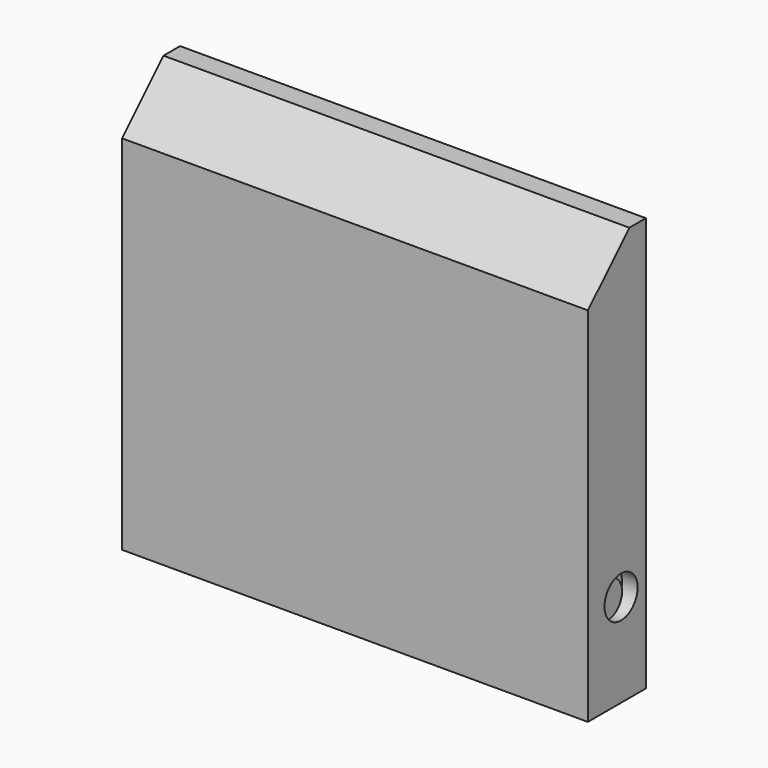
from build123d import *

# Parameters (mm, degrees)
F0_W         = 41
F0_H         = 30
F1_DEPTH     = 6
F2_T         = -2
F3_W         = 2
F3_H         = 2
F4_DEPTH     = 10
F5_R         = 1.75
F6_DEPTH     = 1
F7_R         = 1.75
F8_DEPTH     = 1
F9_W         = 45
F9_H         = 40
F10_DEPTH    = 7
F11_SIZE     = 5
F12_T        = -1.5
F13_T1_DEPTH = 66.7168298797
F16_DEPTH    = 1.5
F17_R        = 2
F18_DEPTH    = 25
F19_R        = 2
F20_DEPTH    = 25
F21_DEPTH    = 2
F22_W        = 14
F22_H        = 12
F22_W_2      = 2
F22_H_2      = 2
F23_DEPTH    = 8


# Not quite as in the source:
# - a fillet or chamfer that OpenCascade refuses, or shapes differently, is made with other operations: its cross-section is extruded or revolved along the edge and cut away or added
# - a feature names something its author has since deleted; it is built from what else it names


with BuildPart() as f1:
    # F0 (on Front) → F1 (new body)
    with BuildSketch(Plane.XZ):
        with Locations((0.5, 0)):
            Rectangle(F0_W, F0_H)
    extrude(amount=F1_DEPTH)

    # F2
    f2_openings = [f1.faces().sort_by_distance(p)[0] for p in [
        (0.5, -6, 0),
    ]]
    offset(amount=F2_T, openings=f2_openings)

    # F3 (on face) → F4 (cut)
    with BuildSketch(Plane.XZ):
        with Locations((-3, -2)):
            Rectangle(F3_W, F3_H)
        with Locations((3, -2)):
            Rectangle(F3_W, F3_H)
        with Locations((3, 2)):
            Rectangle(F3_W, F3_H)
        with Locations((-3, 2)):
            Rectangle(F3_W, F3_H)
    extrude(amount=F4_DEPTH, mode=Mode.SUBTRACT)

    # F5 (on face) → F6 (join)
    with BuildSketch(Plane.YZ.offset(21)):
        with Locations((-4, -11)):
            Circle(F5_R)
    extrude(amount=F6_DEPTH)

    # F7 (on face) → F8 (join)
    with BuildSketch(Plane(origin=(-20, 0, 0), x_dir=(0, -1, 0), z_dir=(-1, 0, 0))):
        with Locations((4, -11)):
            Circle(F7_R)
    extrude(amount=F8_DEPTH)

    # F13: chamfer of 5 on 1 edges, made by hand

    # F13_s2 → F13_t1 (cut)
    with BuildSketch(Plane.YZ.offset(-32.8584149398)):
        Polygon((-1, 15), (-6, 10), (-6, 15), align=None)
    extrude(amount=F13_T1_DEPTH, mode=Mode.SUBTRACT)

    # F22 (on face) → F23 (join)
    with BuildSketch(Plane.XZ.offset(2)):
        Rectangle(F22_W, F22_H)
        with Locations((-3, -2)):
            Rectangle(F22_W_2, F22_H_2, mode=Mode.SUBTRACT)
        with Locations((3, -2)):
            Rectangle(F22_W_2, F22_H_2, mode=Mode.SUBTRACT)
        with Locations((-3, 2)):
            Rectangle(F22_W_2, F22_H_2, mode=Mode.SUBTRACT)
        with Locations((3, 2)):
            Rectangle(F22_W_2, F22_H_2, mode=Mode.SUBTRACT)
    extrude(amount=-F23_DEPTH)


with BuildPart() as f10:
    # F9 (on Front) → F10 (new body)
    with BuildSketch(Plane.XZ):
        Rectangle(F9_W, F9_H)
    extrude(amount=F10_DEPTH)

    # F11
    f11_edges = [f10.edges().sort_by_distance(p)[0] for p in [
        (0, -7, 20),
    ]]
    chamfer(f11_edges, length=F11_SIZE)

    # F12
    f12_openings = [f10.faces().sort_by_distance(p)[0] for p in [
        (0, 0, 0),
    ]]
    offset(amount=F12_T, openings=f12_openings)

    # F15 (on offset) → F16 (join)
    with BuildSketch(Plane(origin=(0, -4, 0), x_dir=(-1, 0, 0), z_dir=(0, 1, 0))):
        with BuildLine():
            Line((-10, -18.5), (10, -18.5))
            Line((10, -18.5), (3.7921958509, 0))
            ThreePointArc((3.7921958509, 0), (0, 2.7275022088), (-3.7921958509, 0))
            Line((-3.7921958509, 0), (-10, -18.5))
        make_face()
    extrude(amount=F16_DEPTH)

    # F17 (on face) → F18 (cut)
    with BuildSketch(Plane.YZ.offset(-21)):
        with Locations((-3, -11)):
            Circle(F17_R)
    extrude(amount=-F18_DEPTH, mode=Mode.SUBTRACT)

    # F19 (on face) → F20 (cut)
    with BuildSketch(Plane(origin=(21, 0, 0), x_dir=(0, -1, 0), z_dir=(-1, 0, 0))):
        with Locations((3, -11)):
            Circle(F19_R)
    extrude(amount=-F20_DEPTH, mode=Mode.SUBTRACT)

    # F21 (add): a face of the model
    f21_faces = [f10.faces().sort_by_distance(p)[0] for p in [
        (0, -0.4235858827, -18.5),
    ]]
    extrude(f21_faces, amount=F21_DEPTH)


solid = Compound([f1.part, f10.part])
